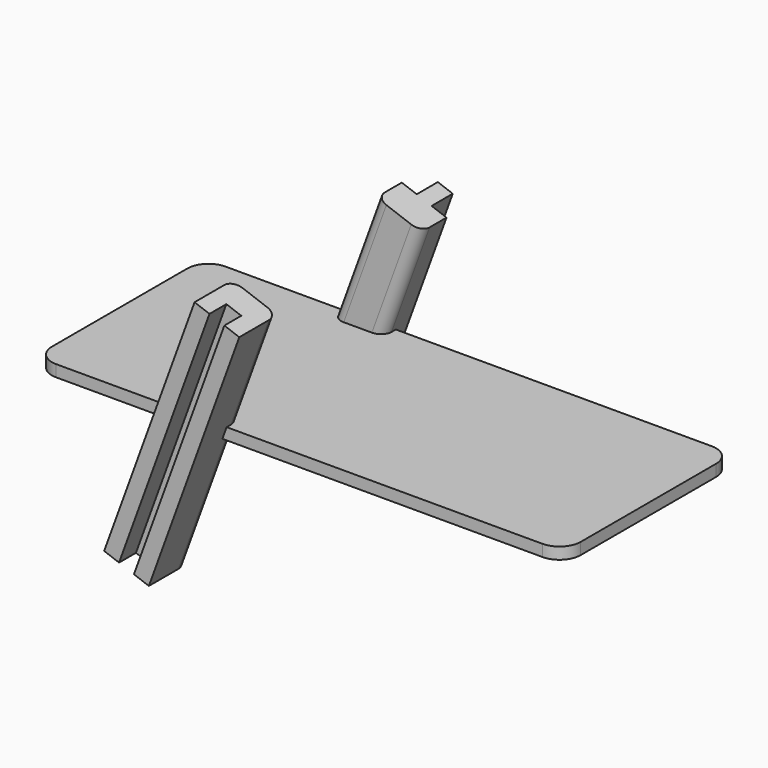
from build123d import *

# Parameters (mm, degrees)
F0_W          = 30.6458014898
F0_H          = 40
F0_W_2        = 69.3541985102
F1_DEPTH      = 2.2
F4_DEPTH      = 25
F4_DEPTH_BACK = 25
F5_R          = 4
F6_R          = 2


# Not quite as in the source:
# - a feature names something its author has since deleted; it is built from what else it names


with BuildPart() as f1:
    # F0 (on Top) → F1 (new body)
    with BuildSketch(Plane.XY):
        with Locations((-27.8972219743, -2.6114098728)):
            Rectangle(F0_W, F0_H)
        with Locations((22.1027780257, -2.6114098728)):
            Rectangle(F0_W_2, F0_H)
    extrude(amount=F1_DEPTH)

    # F3 (on line) → F4 (join, two sides)
    with BuildSketch(Plane(origin=(-1.4709161628, 0, -4.0413089432), x_dir=(0.9396926208, 0, -0.3420201433), z_dir=(-0.3420201433, 0, -0.9396926208))) as f4_sk:
        Polygon((-7.3159968707, -20.3885901272), (-7.3159968707, -14.3885901272), (-11.8159968707, -14.3885901272), (-11.8159968707, -25.3885901272), (-10.3159968707, -25.3885901272), (-10.3159968707, -20.3885901272), align=None)
        Polygon((-11.8159968707, 19.6114098728), (-7.3159968707, 19.6114098728), (-7.3159968707, 28.6114098728), (-10.3159968707, 28.6114098728), (-10.3159968707, 24.6114098728), (-11.8159968707, 24.6114098728), align=None)
        Polygon((-11.8159968707, -25.3885901272), (-11.8159968707, -14.3885901272), (-16.3159968707, -14.3885901272), (-16.3159968707, -20.3885901272), (-13.3159968707, -20.3885901272), (-13.3159968707, -25.3885901272), align=None)
        Polygon((-16.3159968707, 19.6114098728), (-11.8159968707, 19.6114098728), (-11.8159968707, 24.6114098728), (-13.3159968707, 24.6114098728), (-13.3159968707, 28.6114098728), (-16.3159968707, 28.6114098728), align=None)
    extrude(amount=F4_DEPTH)
    extrude(f4_sk.sketch, amount=-F4_DEPTH_BACK)

    # F5
    f5_edges = [f1.edges().sort_by_distance(p)[0] for p in [
        (-43.220123, 17.38859, 1.1),
        (-43.220123, -22.61141, 1.1),
        (56.779877, -22.61141, 1.1),
        (56.779877, 17.38859, 1.1),
    ]]
    fillet(f5_edges, radius=F5_R)

    # F6
    f6_edges = [f1.edges().sort_by_distance(p)[0] for p in [
        (-3.389994, -19.61141, 12.076612),
        (-12.407411, -19.61141, 13.615703),
        (-3.389994, 14.38859, 12.076612),
        (-12.340865, 14.38859, -12.515703),
        (-12.407411, 14.38859, 13.615703),
        (-21.358281, 14.38859, -10.976612),
        (-21.358281, -19.61141, -10.976612),
        (-12.340865, -19.61141, -12.515703),
    ]]
    fillet(f6_edges, radius=F6_R)


solid = f1.part
